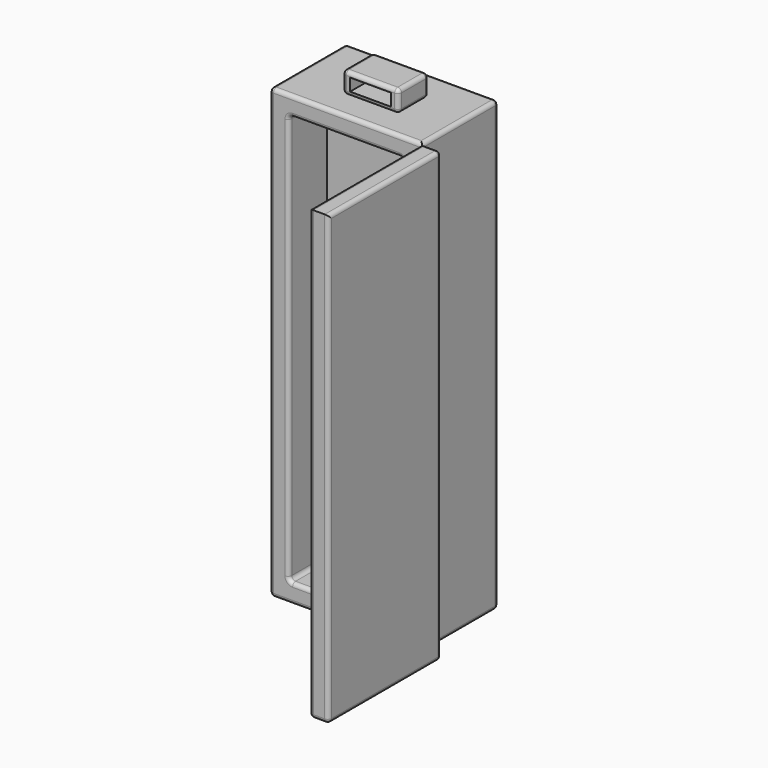
from build123d import *

# Parameters (mm, degrees)
F0_W      = 203.2
F0_H      = 597.2488436915
F1_DEPTH  = 127
F2_T      = -25.4
F3_W      = 152.4
F3_H      = 546.4488436915
F4_DEPTH  = 37.5265
F5_W      = 187.7573173046
F5_H      = 597.2488436915
F6_DEPTH  = 25.4
F7_W      = 74.9618187547
F7_H      = 50.8669428527
F8_DEPTH  = 28.58041
F9_W      = 56.2481023371
F9_H      = 17.1422362328
F10_DEPTH = 76.2
F11_W     = 74.5156109333
F11_H     = 50.4207462072
F12_DEPTH = 28.575
F13_W     = 54.5512109333
F13_H     = 16.5354
F14_DEPTH = 76.2
F15_R     = 5.08
F16_R     = 5.08
F17_R     = 5.08
F17_2_R   = 5.08
F18_R     = 5.08


with BuildPart() as f1:
    # F0 (on Front) → F1 (new body)
    with BuildSketch(Plane.XZ):
        with Locations((70.5637605861, -202.6224955916)):
            Rectangle(F0_W, F0_H)
    extrude(amount=F1_DEPTH)

    # F2
    f2_openings = [f1.faces().sort_by_distance(p)[0] for p in [
        (70.563761, -127, -202.622496),
    ]]
    offset(amount=F2_T, openings=f2_openings)

    # F17
    f17_edges = [f1.edges().sort_by_distance(p)[0] for p in [
        (-31.036239, -63.5, 96.001926),
        (172.163761, -63.5, 96.001926),
        (70.563761, -127, 96.001926),
        (70.563761, 0, 96.001926),
        (-31.036239, 0, -202.622496),
        (-31.036239, -127, -202.622496),
        (70.563761, 0, -501.246917),
        (-31.036239, -63.5, -501.246917),
        (172.163761, -63.5, -501.246917),
        (70.563761, -127, -501.246917),
        (172.163761, 0, -202.622496),
    ]]
    fillet(f17_edges, radius=F17_R)

    # F18
    f18_edges = [f1.edges().sort_by_distance(p)[0] for p in [
        (70.563761, -127, 70.601926),
        (146.763761, -127, -202.622496),
        (-5.636239, -127, -202.622496),
        (70.563761, -127, -475.846917),
        (146.763761, -76.2, -475.846917),
        (-5.636239, -76.2, -475.846917),
        (-5.636239, -76.2, 70.601926),
        (146.763761, -76.2, 70.601926),
    ]]
    fillet(f18_edges, radius=F18_R)


with BuildPart() as f4:
    # F3 (on face) → F4 (new body)
    with BuildSketch(Plane.XZ.offset(25.4)):
        with Locations((70.5637605861, -202.6224955916)):
            Rectangle(F3_W, F3_H)
    extrude(amount=F4_DEPTH)


with BuildPart() as f6:
    # F5 (on face) → F6 (new body)
    with BuildSketch(Plane.YZ.offset(172.1637605861)):
        with Locations((-220.8786586523, -202.6224955916)):
            Rectangle(F5_W, F5_H)
    extrude(amount=F6_DEPTH)

    # F17#2
    f17_2_edges = [f6.edges().sort_by_distance(p)[0] for p in [
        (172.163761, -220.878659, -501.246917),
        (172.163761, -220.878659, 96.001926),
        (172.163761, -314.757317, -202.622496),
        (184.863761, -127, 96.001926),
        (197.563761, -127, -202.622496),
        (197.563761, -220.878659, 96.001926),
        (197.563761, -314.757317, -202.622496),
        (197.563761, -220.878659, -501.246917),
        (184.863761, -314.757317, -501.246917),
        (184.863761, -127, -501.246917),
    ]]
    fillet(f17_2_edges, radius=F17_2_R)


with BuildPart() as f8:
    # F7 (on face) → F8 (new body)
    with BuildSketch(Plane(origin=(0, 0, -501.2469174374), x_dir=(1, 0, 0), z_dir=(0, 0, -1))):
        with Locations((74.7372247279, 66.1760587245)):
            Rectangle(F7_W, F7_H)
    extrude(amount=F8_DEPTH)

    # F9 (on face) → F10 (cut)
    with BuildSketch(Plane.XZ.offset(91.6095301509)):
        with Locations((75.3520485014, -515.8440172672)):
            Rectangle(F9_W, F9_H)
    extrude(amount=-F10_DEPTH, mode=Mode.SUBTRACT)

    # F15
    f15_edges = [f8.edges().sort_by_distance(p)[0] for p in [
        (37.256315, -66.176059, -501.246917),
        (74.737225, -91.60953, -501.246917),
        (112.218134, -66.176059, -501.246917),
        (74.737225, -40.742587, -501.246917),
        (112.218134, -40.742587, -515.537122),
        (112.218134, -91.60953, -515.537122),
        (112.218134, -66.176059, -529.827327),
        (74.737225, -91.60953, -529.827327),
        (37.256315, -66.176059, -529.827327),
        (37.256315, -91.60953, -515.537122),
        (74.737225, -40.742587, -529.827327),
        (37.256315, -40.742587, -515.537122),
    ]]
    fillet(f15_edges, radius=F15_R)


with BuildPart() as f12:
    # F11 (on face) → F12 (new body)
    with BuildSketch(Plane.XY.offset(96.0019262541)):
        with Locations((74.7372284532, -65.9529715776)):
            Rectangle(F11_W, F11_H)
    extrude(amount=F12_DEPTH)

    # F13 (on face) → F14 (cut)
    with BuildSketch(Plane.XZ.offset(91.1633446813)):
        with Locations((74.7372284532, 110.2894262541)):
            Rectangle(F13_W, F13_H)
    extrude(amount=-F14_DEPTH, mode=Mode.SUBTRACT)

    # F16
    f16_edges = [f12.edges().sort_by_distance(p)[0] for p in [
        (111.995034, -91.163345, 110.289426),
        (74.737228, -91.163345, 96.001926),
        (74.737228, -91.163345, 124.576926),
        (37.479423, -91.163345, 110.289426),
        (37.479423, -65.952972, 96.001926),
        (37.479423, -65.952972, 124.576926),
        (111.995034, -65.952972, 124.576926),
        (74.737228, -40.742598, 124.576926),
        (111.995034, -65.952972, 96.001926),
        (111.995034, -40.742598, 110.289426),
        (37.479423, -40.742598, 110.289426),
        (74.737228, -40.742598, 96.001926),
    ]]
    fillet(f16_edges, radius=F16_R)


solid = Compound([f1.part, f4.part, f6.part, f8.part, f12.part])
